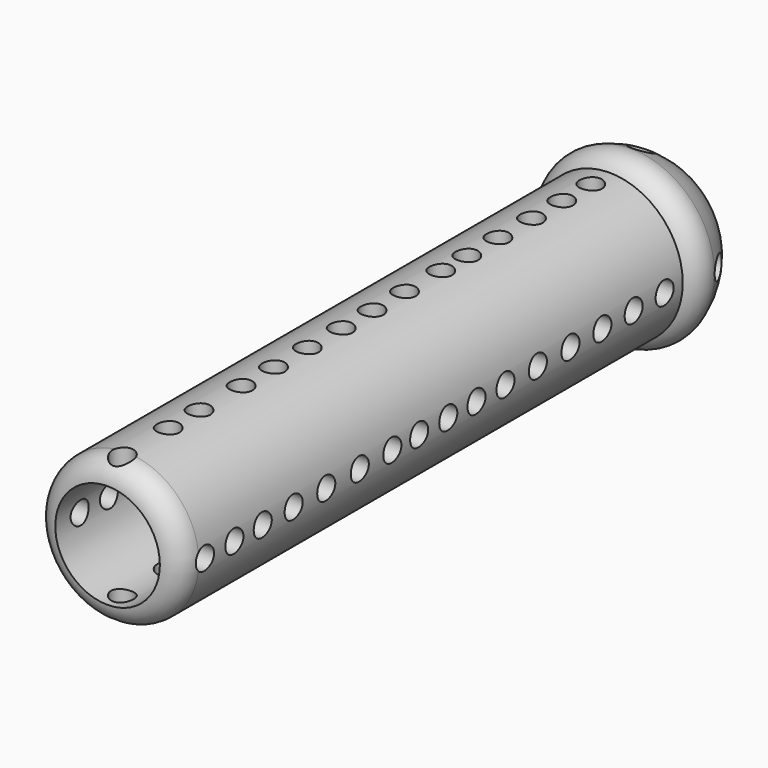
from build123d import *

# Parameters (mm, degrees)
F0_R       = 4.445
F0_R_2     = 3.175
F1_DEPTH   = 38.1
F4_DEPTH   = 38.1
F6_D       = 1.3716
F6_DEPTH   = 5.335
F8_D       = 1.3716
F10_D      = 1.3716
F10_DEPTH  = 5.335
F11_D      = 1.3716
F12_D      = 1.3716
F12_DEPTH  = 5.335
F13_D      = 1.3716
F15_D      = 1.3716
F15_DEPTH  = 5.335
F16_D      = 1.3716
F18_D      = 1.3716
F18_DEPTH  = 5.335
F19_D      = 1.3716
F21_D      = 1.3716
F21_DEPTH  = 5.335
F22_D      = 1.3716
F24_D      = 1.3716
F24_DEPTH  = 5.335
F25_D      = 1.3716
F27_D      = 1.3716
F27_DEPTH  = 5.335
F28_D      = 1.3716
F30_D      = 1.3716
F30_DEPTH  = 5.335
F31_D      = 1.3716
F33_D      = 1.3716
F33_DEPTH  = 5.335
F34_D      = 1.3716
F36_D      = 1.3716
F36_DEPTH  = 5.335
F37_D      = 1.3716
F39_D      = 1.3716
F39_DEPTH  = 5.335
F40_D      = 1.3716
F42_D      = 1.3716
F42_DEPTH  = 5.335
F43_D      = 1.3716
F45_D      = 1.3716
F45_DEPTH  = 5.335
F46_D      = 1.3716
F48_D      = 1.3716
F48_DEPTH  = 5.335
F49_D      = 1.3716
F51_D      = 1.3716
F51_DEPTH  = 5.335
F52_D      = 1.3716
F54_D      = 1.3716
F56_D      = 1.3716
F56_DEPTH  = 5.335
F57_D      = 1.3716
F59_D      = 1.3716
F59_DEPTH  = 5.335
F60_D      = 1.3716
F62_D      = 1.3716
F62_DEPTH  = 5.335
F63_D      = 1.3716
F65_D      = 1.3716
F65_DEPTH  = 5.335
F66_D      = 1.3716
F68_D      = 1.3716
F68_DEPTH  = 5.335
F69_D      = 1.3716
F71_D      = 1.3716
F71_DEPTH  = 5.335
F72_D      = 1.3716
F74_D      = 1.3716
F74_DEPTH  = 5.335
F75_D      = 1.3716
F77_D      = 1.3716
F77_DEPTH  = 5.335
F78_D      = 1.3716
F80_D      = 1.3716
F80_DEPTH  = 5.335
F81_D      = 1.3716
F83_D      = 1.3716
F83_DEPTH  = 5.335
F84_D      = 1.3716
F86_D      = 1.3716
F86_DEPTH  = 5.335
F87_D      = 1.3716
F89_D      = 1.3716
F89_DEPTH  = 5.335
F90_D      = 1.3716
F92_D      = 1.3716
F92_DEPTH  = 5.335
F93_D      = 1.3716
F95_D      = 1.3716
F95_DEPTH  = 5.335
F96_D      = 1.3716
F98_D      = 1.3716
F98_DEPTH  = 5.335
F99_D      = 1.3716
F101_D     = 1.3716
F101_DEPTH = 5.335
F102_D     = 1.3716
F104_D     = 1.3716
F104_DEPTH = 5.335
F105_D     = 1.3716


# Not quite as in the source:
# - a fillet or chamfer that OpenCascade refuses, or shapes differently, is made with other operations: its cross-section is extruded or revolved along the edge and cut away or added


with BuildPart() as f1:
    # F0 (on Front) → F1 (new body)
    with BuildSketch(Plane.XZ):
        Circle(F0_R)
        Circle(F0_R_2, mode=Mode.SUBTRACT)
    extrude(amount=F1_DEPTH)

    # F2 (on Top) → F3 (revolve)
    with BuildSketch(Plane.XY):
        with BuildLine():
            Line((0, 0), (5.334, 0))
            ThreePointArc((5.334, 0), (3.7717075708, 3.7717075708), (0, 5.334))
            Line((0, 5.334), (0, 0))
        make_face()
    revolve(axis=Axis((0, 2.667, 0), (0, -1, 0)))

    # F0 (on Front) → F4 (join)
    with BuildSketch(Plane.XZ):
        Circle(F0_R)
        Circle(F0_R_2, mode=Mode.SUBTRACT)
    extrude(amount=F4_DEPTH)

    # F6 (through all, one way)
    with BuildSketch(Plane.YZ):
        with Locations((-1.3715132581, 0)):
            Circle(F6_D / 2)
    extrude(amount=-F6_DEPTH, mode=Mode.SUBTRACT)

    # F8 (through all)
    with Locations(Plane(origin=(0, 0, 0), x_dir=(0, 1, 0), z_dir=(-1, 0, 0))):
        with Locations((-1.3715132581, 0)):
            Hole(F8_D / 2)

    # F10 (through all, one way)
    with BuildSketch(Plane.YZ):
        with Locations((-6.0971285944, 0)):
            Circle(F10_D / 2)
    extrude(amount=-F10_DEPTH, mode=Mode.SUBTRACT)

    # F11 (through all)
    with Locations(Plane(origin=(0, 0, 0), x_dir=(0, 1, 0), z_dir=(-1, 0, 0))):
        with Locations((-6.0971285944, 0)):
            Hole(F11_D / 2)

    # F12 (through all, one way)
    with BuildSketch(Plane.YZ):
        with Locations((-3.7209431116, 0)):
            Circle(F12_D / 2)
    extrude(amount=-F12_DEPTH, mode=Mode.SUBTRACT)

    # F13 (through all)
    with Locations(Plane(origin=(0, 0, 0), x_dir=(0, 1, 0), z_dir=(-1, 0, 0))):
        with Locations((-3.7209431116, 0)):
            Hole(F13_D / 2)

    # F15 (through all, one way)
    with BuildSketch(Plane.YZ):
        with Locations((-8.5155256093, 0)):
            Circle(F15_D / 2)
    extrude(amount=-F15_DEPTH, mode=Mode.SUBTRACT)

    # F16 (through all)
    with Locations(Plane(origin=(0, 0, 0), x_dir=(0, 1, 0), z_dir=(-1, 0, 0))):
        with Locations((-8.5155256093, 0)):
            Hole(F16_D / 2)

    # F18 (through all, one way)
    with BuildSketch(Plane.YZ):
        with Locations((-10.9913162982, 0)):
            Circle(F18_D / 2)
    extrude(amount=-F18_DEPTH, mode=Mode.SUBTRACT)

    # F19 (through all)
    with Locations(Plane(origin=(0, 0, 0), x_dir=(0, 1, 0), z_dir=(-1, 0, 0))):
        with Locations((-10.9913162982, 0)):
            Hole(F19_D / 2)

    # F21 (through all, one way)
    with BuildSketch(Plane.YZ):
        with Locations((-13.4483510628, 0)):
            Circle(F21_D / 2)
    extrude(amount=-F21_DEPTH, mode=Mode.SUBTRACT)

    # F22 (through all)
    with Locations(Plane(origin=(0, 0, 0), x_dir=(0, 1, 0), z_dir=(-1, 0, 0))):
        with Locations((-13.4483510628, 0)):
            Hole(F22_D / 2)

    # F24 (through all, one way)
    with BuildSketch(Plane.YZ):
        with Locations((-15.6512405019, 0)):
            Circle(F24_D / 2)
    extrude(amount=-F24_DEPTH, mode=Mode.SUBTRACT)

    # F25 (through all)
    with Locations(Plane(origin=(0, 0, 0), x_dir=(0, 1, 0), z_dir=(-1, 0, 0))):
        with Locations((-15.6512405019, 0)):
            Hole(F25_D / 2)

    # F27 (through all, one way)
    with BuildSketch(Plane.YZ):
        with Locations((-17.795778811, 0)):
            Circle(F27_D / 2)
    extrude(amount=-F27_DEPTH, mode=Mode.SUBTRACT)

    # F28 (through all)
    with Locations(Plane(origin=(0, 0, 0), x_dir=(0, 1, 0), z_dir=(-1, 0, 0))):
        with Locations((-17.795778811, 0)):
            Hole(F28_D / 2)

    # F30 (through all, one way)
    with BuildSketch(Plane.YZ):
        with Locations((-20.0037695467, 0)):
            Circle(F30_D / 2)
    extrude(amount=-F30_DEPTH, mode=Mode.SUBTRACT)

    # F31 (through all)
    with Locations(Plane(origin=(0, 0, 0), x_dir=(0, 1, 0), z_dir=(-1, 0, 0))):
        with Locations((-20.0037695467, 0)):
            Hole(F31_D / 2)

    # F33 (through all, one way)
    with BuildSketch(Plane.YZ):
        with Locations((-22.0396984369, 0)):
            Circle(F33_D / 2)
    extrude(amount=-F33_DEPTH, mode=Mode.SUBTRACT)

    # F34 (through all)
    with Locations(Plane(origin=(0, 0, 0), x_dir=(0, 1, 0), z_dir=(-1, 0, 0))):
        with Locations((-22.0396984369, 0)):
            Hole(F34_D / 2)

    # F36 (through all, one way)
    with BuildSketch(Plane.YZ):
        with Locations((-24.5118960738, 0)):
            Circle(F36_D / 2)
    extrude(amount=-F36_DEPTH, mode=Mode.SUBTRACT)

    # F37 (through all)
    with Locations(Plane(origin=(0, 0, 0), x_dir=(0, 1, 0), z_dir=(-1, 0, 0))):
        with Locations((-24.5118960738, 0)):
            Hole(F37_D / 2)

    # F39 (through all, one way)
    with BuildSketch(Plane.YZ):
        with Locations((-27.0568039268, 0)):
            Circle(F39_D / 2)
    extrude(amount=-F39_DEPTH, mode=Mode.SUBTRACT)

    # F40 (through all)
    with Locations(Plane(origin=(0, 0, 0), x_dir=(0, 1, 0), z_dir=(-1, 0, 0))):
        with Locations((-27.0568039268, 0)):
            Hole(F40_D / 2)

    # F42 (through all, one way)
    with BuildSketch(Plane.YZ):
        with Locations((-29.5290034264, 0)):
            Circle(F42_D / 2)
    extrude(amount=-F42_DEPTH, mode=Mode.SUBTRACT)

    # F43 (through all)
    with Locations(Plane(origin=(0, 0, 0), x_dir=(0, 1, 0), z_dir=(-1, 0, 0))):
        with Locations((-29.5290034264, 0)):
            Hole(F43_D / 2)

    # F45 (through all, one way)
    with BuildSketch(Plane.YZ):
        with Locations((-31.8767800927, 0)):
            Circle(F45_D / 2)
    extrude(amount=-F45_DEPTH, mode=Mode.SUBTRACT)

    # F46 (through all)
    with Locations(Plane(origin=(0, 0, 0), x_dir=(0, 1, 0), z_dir=(-1, 0, 0))):
        with Locations((-31.8767800927, 0)):
            Hole(F46_D / 2)

    # F48 (through all, one way)
    with BuildSketch(Plane.YZ):
        with Locations((-34.0286567807, 0)):
            Circle(F48_D / 2)
    extrude(amount=-F48_DEPTH, mode=Mode.SUBTRACT)

    # F49 (through all)
    with Locations(Plane(origin=(0, 0, 0), x_dir=(0, 1, 0), z_dir=(-1, 0, 0))):
        with Locations((-34.0286567807, 0)):
            Hole(F49_D / 2)

    # F51 (through all, one way)
    with BuildSketch(Plane.YZ):
        with Locations((-36.2560003996, 0)):
            Circle(F51_D / 2)
    extrude(amount=-F51_DEPTH, mode=Mode.SUBTRACT)

    # F52 (through all)
    with Locations(Plane(origin=(0, 0, 0), x_dir=(0, 1, 0), z_dir=(-1, 0, 0))):
        with Locations((-36.2560003996, 0)):
            Hole(F52_D / 2)

    # F54 (through all)
    with Locations(Plane.XZ):
        with Locations((0, 0)):
            Hole(F54_D / 2)

    # F56 (through all, one way)
    with BuildSketch(Plane.YZ):
        with Locations((2.3186756057, 0)):
            Circle(F56_D / 2)
    extrude(amount=-F56_DEPTH, mode=Mode.SUBTRACT)

    # F57 (through all)
    with Locations(Plane(origin=(0, 0, 0), x_dir=(0, 1, 0), z_dir=(-1, 0, 0))):
        with Locations((2.3186756057, 0)):
            Hole(F57_D / 2)

    # F59 (through all, one way)
    with BuildSketch(Plane.XY):
        with Locations((0, -1.4289842018)):
            Circle(F59_D / 2)
    extrude(amount=-F59_DEPTH, mode=Mode.SUBTRACT)

    # F60 (through all)
    with Locations(Plane(origin=(0, 0, 0), x_dir=(1, 0, 0), z_dir=(0, 0, -1))):
        with Locations((0, 1.4289842018)):
            Hole(F60_D / 2)

    # F62 (through all, one way)
    with BuildSketch(Plane.XY):
        with Locations((0, -3.6302781218)):
            Circle(F62_D / 2)
    extrude(amount=-F62_DEPTH, mode=Mode.SUBTRACT)

    # F63 (through all)
    with Locations(Plane(origin=(0, 0, 0), x_dir=(1, 0, 0), z_dir=(0, 0, -1))):
        with Locations((0, 3.6302781218)):
            Hole(F63_D / 2)

    # F65 (through all, one way)
    with BuildSketch(Plane.XY):
        with Locations((0, -5.928453058)):
            Circle(F65_D / 2)
    extrude(amount=-F65_DEPTH, mode=Mode.SUBTRACT)

    # F66 (through all)
    with Locations(Plane(origin=(0, 0, 0), x_dir=(1, 0, 0), z_dir=(0, 0, -1))):
        with Locations((0, 5.928453058)):
            Hole(F66_D / 2)

    # F68 (through all, one way)
    with BuildSketch(Plane.XY):
        with Locations((0, -8.4759704769)):
            Circle(F68_D / 2)
    extrude(amount=-F68_DEPTH, mode=Mode.SUBTRACT)

    # F69 (through all)
    with Locations(Plane(origin=(0, 0, 0), x_dir=(1, 0, 0), z_dir=(0, 0, -1))):
        with Locations((0, 8.4759704769)):
            Hole(F69_D / 2)

    # F71 (through all, one way)
    with BuildSketch(Plane.XY):
        with Locations((0, -10.8355125412)):
            Circle(F71_D / 2)
    extrude(amount=-F71_DEPTH, mode=Mode.SUBTRACT)

    # F72 (through all)
    with Locations(Plane(origin=(0, 0, 0), x_dir=(1, 0, 0), z_dir=(0, 0, -1))):
        with Locations((0, 10.8355125412)):
            Hole(F72_D / 2)

    # F74 (through all, one way)
    with BuildSketch(Plane.XY):
        with Locations((0, -12.8123224325)):
            Circle(F74_D / 2)
    extrude(amount=-F74_DEPTH, mode=Mode.SUBTRACT)

    # F75 (through all)
    with Locations(Plane(origin=(0, 0, 0), x_dir=(1, 0, 0), z_dir=(0, 0, -1))):
        with Locations((0, 12.8123224325)):
            Hole(F75_D / 2)

    # F77 (through all, one way)
    with BuildSketch(Plane.XY):
        with Locations((0, -15.5655970052)):
            Circle(F77_D / 2)
    extrude(amount=-F77_DEPTH, mode=Mode.SUBTRACT)

    # F78 (through all)
    with Locations(Plane(origin=(0, 0, 0), x_dir=(1, 0, 0), z_dir=(0, 0, -1))):
        with Locations((0, 15.5655970052)):
            Hole(F78_D / 2)

    # F80 (through all, one way)
    with BuildSketch(Plane.XY):
        with Locations((0, -18.0249679834)):
            Circle(F80_D / 2)
    extrude(amount=-F80_DEPTH, mode=Mode.SUBTRACT)

    # F81 (through all)
    with Locations(Plane(origin=(0, 0, 0), x_dir=(1, 0, 0), z_dir=(0, 0, -1))):
        with Locations((0, 18.0249679834)):
            Hole(F81_D / 2)

    # F83 (through all, one way)
    with BuildSketch(Plane.XY):
        with Locations((0, -20.3684661537)):
            Circle(F83_D / 2)
    extrude(amount=-F83_DEPTH, mode=Mode.SUBTRACT)

    # F84 (through all)
    with Locations(Plane(origin=(0, 0, 0), x_dir=(1, 0, 0), z_dir=(0, 0, -1))):
        with Locations((0, 20.3684661537)):
            Hole(F84_D / 2)

    # F86 (through all, one way)
    with BuildSketch(Plane.XY):
        with Locations((0, -25.5097380026)):
            Circle(F86_D / 2)
    extrude(amount=-F86_DEPTH, mode=Mode.SUBTRACT)

    # F87 (through all)
    with Locations(Plane(origin=(0, 0, 0), x_dir=(1, 0, 0), z_dir=(0, 0, -1))):
        with Locations((0, 25.5097380026)):
            Hole(F87_D / 2)

    # F89 (through all, one way)
    with BuildSketch(Plane.XY):
        with Locations((0, -22.9434985667)):
            Circle(F89_D / 2)
    extrude(amount=-F89_DEPTH, mode=Mode.SUBTRACT)

    # F90 (through all)
    with Locations(Plane(origin=(0, 0, 0), x_dir=(1, 0, 0), z_dir=(0, 0, -1))):
        with Locations((0, 22.9434985667)):
            Hole(F90_D / 2)

    # F92 (through all, one way)
    with BuildSketch(Plane.XY):
        with Locations((0, -27.9648117721)):
            Circle(F92_D / 2)
    extrude(amount=-F92_DEPTH, mode=Mode.SUBTRACT)

    # F93 (through all)
    with Locations(Plane(origin=(0, 0, 0), x_dir=(1, 0, 0), z_dir=(0, 0, -1))):
        with Locations((0, 27.9648117721)):
            Hole(F93_D / 2)

    # F95 (through all, one way)
    with BuildSketch(Plane.XY):
        with Locations((0, -31.161687256)):
            Circle(F95_D / 2)
    extrude(amount=-F95_DEPTH, mode=Mode.SUBTRACT)

    # F96 (through all)
    with Locations(Plane(origin=(0, 0, 0), x_dir=(1, 0, 0), z_dir=(0, 0, -1))):
        with Locations((0, 31.161687256)):
            Hole(F96_D / 2)

    # F98 (through all, one way)
    with BuildSketch(Plane.XY):
        with Locations((0, -33.5011333227)):
            Circle(F98_D / 2)
    extrude(amount=-F98_DEPTH, mode=Mode.SUBTRACT)

    # F99 (through all)
    with Locations(Plane(origin=(0, 0, 0), x_dir=(1, 0, 0), z_dir=(0, 0, -1))):
        with Locations((0, 33.5011333227)):
            Hole(F99_D / 2)

    # F101 (through all, one way)
    with BuildSketch(Plane.XY):
        with Locations((0, -36.9774252176)):
            Circle(F101_D / 2)
    extrude(amount=-F101_DEPTH, mode=Mode.SUBTRACT)

    # F102 (through all)
    with Locations(Plane(origin=(0, 0, 0), x_dir=(1, 0, 0), z_dir=(0, 0, -1))):
        with Locations((0, 36.9774252176)):
            Hole(F102_D / 2)

    # F104 (through all, one way)
    with BuildSketch(Plane.XY):
        with Locations((0, 2.4021529613)):
            Circle(F104_D / 2)
    extrude(amount=-F104_DEPTH, mode=Mode.SUBTRACT)

    # F105 (through all)
    with Locations(Plane(origin=(0, 0, 0), x_dir=(1, 0, 0), z_dir=(0, 0, -1))):
        with Locations((0, -2.4021529613)):
            Hole(F105_D / 2)

    # F106: fillet of radius 1.3716 on 1 edges, made by hand

    # F106_s1 → F106_t2 (revolve, cut)
    with BuildSketch(Plane.XY):
        with BuildLine():
            ThreePointArc((4.445, 0), (5.0520113475, 0.6923790028), (5.0843961538, 1.6125978267))
            ThreePointArc((5.0843961538, 1.6125978267), (5.2712296993, 0.8159003969), (5.334, 0))
            Line((5.334, 0), (4.445, 0))
        make_face()
    revolve(axis=Axis((0, 0, 0), (0, -1, 0)), mode=Mode.SUBTRACT)

    # F107: fillet of radius 1.3716 on 1 edges, made by hand

    # F107_s1 → F107_t2 (revolve, cut)
    with BuildSketch(Plane.XY):
        with BuildLine():
            ThreePointArc((4.445, -36.732168139), (4.078547034, -37.665423731), (3.175, -38.1))
            Line((3.175, -38.1), (4.445, -38.1))
            Line((4.445, -38.1), (4.445, -36.732168139))
        make_face()
    revolve(axis=Axis((0, -38.1, 0), (0, -1, 0)), mode=Mode.SUBTRACT)


solid = f1.part
